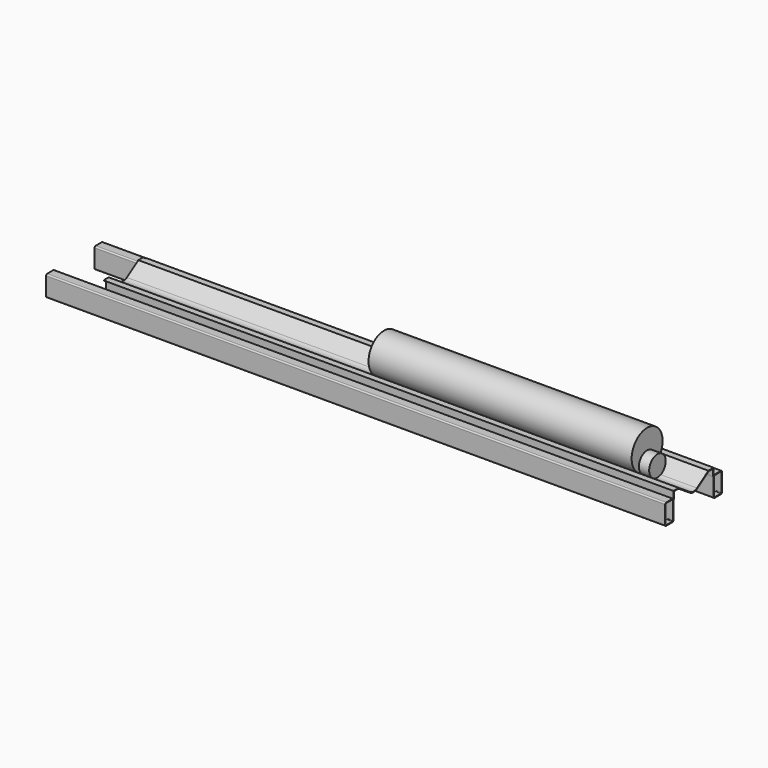
from build123d import *

# Parameters (mm, degrees)
F1_DEPTH = 6096
F2_DEPTH = 5588
F3_START = -355.6
F3_DEPTH = 2692.4
F4_START = -457.2
F4_DEPTH = 2590.8
F7_DEPTH = 25.4


# Not quite as in the source:
# - a feature names something its author has since deleted; it is built from what else it names


with BuildPart() as f1:
    # F0 (on Right) → F1 (new body)
    with BuildSketch(Plane.YZ):
        with BuildLine():
            Line((-278.751844046, 57.15), (-336.55, 57.15))
            ThreePointArc((-336.55, 57.15), (-345.5302561211, 53.4302561211), (-349.25, 44.45))
            Line((-349.25, 44.45), (-349.25, -133.35))
            ThreePointArc((-349.25, -133.35), (-345.5302561211, -142.3302561211), (-336.55, -146.05))
            Line((-336.55, -146.05), (-260.35, -146.05))
            ThreePointArc((-260.35, -146.05), (-251.3697438789, -142.3302561211), (-247.65, -133.35))
            Line((-247.65, -133.35), (-247.65, 44.45))
            ThreePointArc((-247.65, 44.45), (-251.3697438789, 53.4302561211), (-260.35, 57.15))
            Line((-260.35, 57.15), (-268.1402802436, 57.15))
            Line((-268.1402802436, 57.15), (-269.3472818438, 57.15))
            Line((-269.3472818438, 57.15), (-278.751844046, 57.15))
        make_face()
        with BuildLine():
            ThreePointArc((-342.9, 44.45), (-341.0401280605, 48.9401280605), (-336.55, 50.8))
            Line((-336.55, 50.8), (-260.35, 50.8))
            ThreePointArc((-260.35, 50.8), (-255.8598719395, 48.9401280605), (-254, 44.45))
            Line((-254, 44.45), (-254, -133.35))
            ThreePointArc((-254, -133.35), (-255.8598719395, -137.8401280605), (-260.35, -139.7))
            Line((-260.35, -139.7), (-336.55, -139.7))
            ThreePointArc((-336.55, -139.7), (-341.0401280605, -137.8401280605), (-342.9, -133.35))
            Line((-342.9, -133.35), (-342.9, 44.45))
        make_face(mode=Mode.SUBTRACT)
    extrude(amount=-F1_DEPTH)


with BuildPart() as f1b:
    # F0 (on Right) → F1, piece 2 (new body)
    with BuildSketch(Plane.YZ):
        with BuildLine():
            ThreePointArc((260.35, 57.15), (251.3697438789, 53.4302561211), (247.65, 44.45))
            Line((247.65, 44.45), (247.65, -133.35))
            ThreePointArc((247.65, -133.35), (251.3697438789, -142.3302561211), (260.35, -146.05))
            Line((260.35, -146.05), (336.55, -146.05))
            ThreePointArc((336.55, -146.05), (345.5302561211, -142.3302561211), (349.25, -133.35))
            Line((349.25, -133.35), (349.25, 44.45))
            ThreePointArc((349.25, 44.45), (345.5302561211, 53.4302561211), (336.55, 57.15))
            Line((336.55, 57.15), (260.35, 57.15))
        make_face()
        with BuildLine():
            Line((260.35, 50.8), (336.55, 50.8))
            ThreePointArc((336.55, 50.8), (341.0401280605, 48.9401280605), (342.9, 44.45))
            Line((342.9, 44.45), (342.9, -133.35))
            ThreePointArc((342.9, -133.35), (341.0401280605, -137.8401280605), (336.55, -139.7))
            Line((336.55, -139.7), (260.35, -139.7))
            ThreePointArc((260.35, -139.7), (255.8598719395, -137.8401280605), (254, -133.35))
            Line((254, -133.35), (254, 44.45))
            ThreePointArc((254, 44.45), (255.8598719395, 48.9401280605), (260.35, 50.8))
        make_face(mode=Mode.SUBTRACT)
    extrude(amount=-F1_DEPTH)


with BuildPart() as f2:
    # F0 (on Right) → F2 (new body)
    with BuildSketch(Plane.YZ):
        with BuildLine():
            Line((-247.65, 120.65), (-247.65, 44.45))
            Line((-247.65, 44.45), (-241.3, 44.45))
            Line((-241.3, 44.45), (-241.3, 114.3))
            Line((-241.3, 114.3), (-184.7652837227, 114.3))
            Line((-184.7652837227, 114.3), (-45.4622963682, 22.3882611001))
            ThreePointArc((-45.4622963682, 22.3882611001), (0, 8.7416870594), (45.4622963682, 22.3882611001))
            Line((45.4622963682, 22.3882611001), (184.7652837227, 114.3))
            Line((184.7652837227, 114.3), (241.3, 114.3))
            Line((241.3, 114.3), (241.3, 44.45))
            Line((241.3, 44.45), (247.65, 44.45))
            Line((247.65, 44.45), (247.65, 120.65))
            Line((247.65, 120.65), (182.8591823578, 120.65))
            Line((182.8591823578, 120.65), (104.9129874888, 69.2213088636))
            Line((104.9129874888, 69.2213088636), (55.9535927255, 36.9180309968))
            Line((55.9535927255, 36.9180309968), (41.9651966475, 27.6885246354))
            ThreePointArc((41.9651966475, 27.6885246354), (0, 15.0916870594), (-41.9651966475, 27.6885246354))
            Line((-41.9651966475, 27.6885246354), (-55.9535977541, 36.9180343146))
            Line((-55.9535977541, 36.9180343146), (-104.9129888218, 69.2213097431))
            Line((-104.9129888218, 69.2213097431), (-182.8591823578, 120.65))
            Line((-182.8591823578, 120.65), (-247.65, 120.65))
        make_face()
    extrude(amount=-F2_DEPTH)

    # F6 (on face) → F7 (join)
    with BuildSketch(Plane(origin=(-5588, 0, 0), x_dir=(0, -1, 0), z_dir=(-1, 0, 0))):
        with BuildLine():
            Line((-241.3, 120.65), (-241.3, 114.3))
            Line((-241.3, 114.3), (-184.7652837227, 114.3))
            Line((-184.7652837227, 114.3), (-45.4622963682, 22.3882611001))
            ThreePointArc((-45.4622963682, 22.3882611001), (0, 8.7416870594), (45.4622963682, 22.3882611001))
            Line((45.4622963682, 22.3882611001), (184.7652837227, 114.3))
            Line((184.7652837227, 114.3), (241.3, 114.3))
            Line((241.3, 114.3), (241.3, 120.65))
            Line((241.3, 120.65), (182.8591823578, 120.65))
            Line((182.8591823578, 120.65), (41.9651966475, 27.6885246354))
            ThreePointArc((41.9651966475, 27.6885246354), (0, 15.0916870594), (-41.9651966475, 27.6885246354))
            Line((-41.9651966475, 27.6885246354), (-182.8591823578, 120.65))
            Line((-182.8591823578, 120.65), (-241.3, 120.65))
        make_face()
    extrude(amount=F7_DEPTH)


with BuildPart() as f3:
    # F0 (on Right) → F3 (new body)
    with BuildSketch(Plane.YZ.offset(F3_START)):
        with BuildLine():
            ThreePointArc((-74.8958186051, 53.0696722179), (-65.9212506869, 44.4115211281), (-55.9535977541, 36.9180343146))
            ThreePointArc((-55.9535977541, 36.9180343146), (-3.0123e-06, 20.1222494126), (55.9535927255, 36.9180309968))
            ThreePointArc((55.9535927255, 36.9180309968), (65.9212483948, 44.4115191736), (74.8958186051, 53.0696722179))
            ThreePointArc((74.8958186051, 53.0696722179), (0, 37.7292176485), (-74.8958186051, 53.0696722179))
        make_face()
        with BuildLine():
            ThreePointArc((101.6, 121.7222494126), (-36.8316767859, 216.4111483667), (-74.8958186051, 53.0696722179))
            ThreePointArc((-74.8958186051, 53.0696722179), (0, 37.7292176485), (74.8958186051, 53.0696722179))
            ThreePointArc((74.8958186051, 53.0696722179), (94.6888989541, 84.8905726267), (101.6, 121.7222494126))
        make_face()
    extrude(amount=-F3_DEPTH)


with BuildPart() as f4:
    # F0 (on Right) → F4 (new body)
    with BuildSketch(Plane.YZ.offset(F4_START)):
        with BuildLine():
            ThreePointArc((190.5, 228.2292176485), (-90.2893283546, 395.9733298709), (-104.9129888218, 69.2213097431))
            ThreePointArc((-104.9129888218, 69.2213097431), (-90.2663871868, 60.4727592207), (-74.8958186051, 53.0696722179))
            ThreePointArc((-74.8958186051, 53.0696722179), (-36.8316767859, 216.4111483667), (101.6, 121.7222494126))
            ThreePointArc((101.6, 121.7222494126), (94.6888989541, 84.8905726267), (74.8958186051, 53.0696722179))
            ThreePointArc((74.8958186051, 53.0696722179), (90.2663864837, 60.4727588424), (104.9129874888, 69.2213088636))
            ThreePointArc((104.9129874888, 69.2213088636), (167.7441118439, 137.9398885908), (190.5, 228.2292176485))
        make_face()
        with BuildLine():
            ThreePointArc((101.6, 121.7222494126), (-36.8316767859, 216.4111483667), (-74.8958186051, 53.0696722179))
            ThreePointArc((-74.8958186051, 53.0696722179), (0, 37.7292176485), (74.8958186051, 53.0696722179))
            ThreePointArc((74.8958186051, 53.0696722179), (94.6888989541, 84.8905726267), (101.6, 121.7222494126))
        make_face()
    extrude(amount=-F4_DEPTH)


solid = Compound([f1.part, f1b.part, f2.part, f3.part, f4.part])
